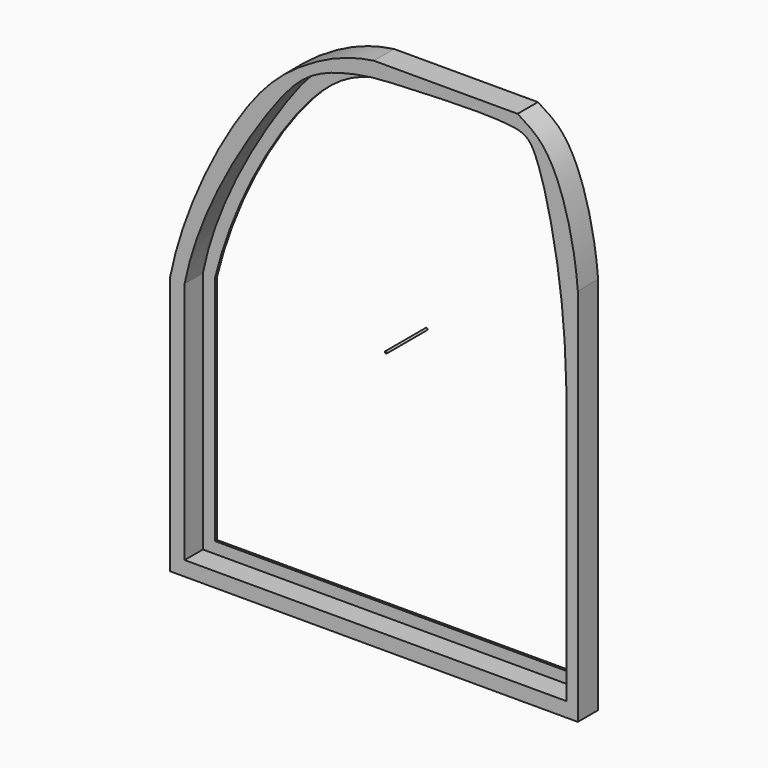
from build123d import *

# Parameters (mm, degrees)
F0_R     = 0.2107517129
F1_DEPTH = 10
F3_DEPTH = 5
F4_DEPTH = 0.5


with BuildPart() as f1:
    # F0 (on Front) → F1 (new body)
    with BuildSketch(Plane.XZ):
        Circle(F0_R)
    extrude(amount=F1_DEPTH)


with BuildPart() as f3:
    # F2 (on Front) → F3 (new body)
    with BuildSketch(Plane.XZ):
        with BuildLine():
            Line((21.9498877709, 46.5069999899), (-6.3801594079, 46.5069999899))
            add(Edge.make_bspline(
                [(-46.5855710208, -4.3176412582), (-44.0025745855, 8.8650835819), (-32.3669471438, 31.5826223404), (-20.8450996019, 41.430559805), (-11.9788710798, 45.7277535437), (-6.3801594079, 46.5069999899)],
                knots=[0, 0, 0, 0, 0.4471722481, 0.7226417186, 1, 1, 1, 1], degree=3))
            Line((-46.5855710208, -4.3176412582), (-46.5855710208, -55.1422825063))
            Line((-46.5855710208, -55.1422825063), (33.8252522051, -55.1422825063))
            Line((33.8252522051, -55.1422825063), (33.8252522051, 3.3716567512))
            add(Edge.make_bspline(
                [(33.8252522051, 3.4864664458), (33.8224510146, 3.4189701607), (33.823496077, 3.4012213221), (33.8252522051, 3.3716567512)],
                knots=[0.9714616128, 0.9714616128, 0.9714616128, 0.9714616128, 1, 1, 1, 1], degree=3))
            Line((33.8252522051, 3.4864664458), (33.8252522051, 19.6025110781))
            add(Edge.make_bspline(
                [(21.9498877709, 46.5069999899), (23.8964492564, 45.3404017708), (29.3341911452, 42.1357952335), (33.1026848595, 28.5809846581), (33.8252522051, 19.6025110781)],
                knots=[0, 0, 0, 0, 0.2303722913, 0.6333427683, 0.6333427683, 0.6333427683, 0.6333427683], degree=3))
        make_face()
        with BuildLine():
            Line((31.6210500896, -52.260261029), (-43.6766035855, -52.260261029))
            Line((-43.6766035855, -52.260261029), (-43.6766035855, -4.3176412582))
            add(Edge.make_bspline(
                [(-43.6766035855, -4.3176412582), (-41.0383021138, 9.0666906176), (-27.9398807539, 30.9156219348), (-18.7479844266, 41.3390835094), (-7.0085331076, 43.5985571671), (-2.215007715, 43.8020735184), (21.2993443911, 44.9657713637), (26.0800513958, 41.7197839808), (31.3102526714, 18.3624746495), (31.5930695379, 3.1075431018), (31.6210500896, -4.3176412582)],
                knots=[0, 0, 0, 0, 0.1942047864, 0.3092342936, 0.40822929, 0.4837495286, 0.6306580628, 0.7017097882, 0.8479049191, 1, 1, 1, 1], degree=3))
            Line((31.6210500896, -4.3176412582), (31.6210500896, -52.260261029))
        make_face(mode=Mode.SUBTRACT)
        with BuildLine():
            Line((33.8252522051, 3.3716567512), (33.8252522051, 3.4864664458))
            add(Edge.make_bspline(
                [(33.8252522051, 3.4864664458), (33.8224510146, 3.4189701607), (33.823496077, 3.4012213221), (33.8252522051, 3.3716567512)],
                knots=[0.9714616128, 0.9714616128, 0.9714616128, 0.9714616128, 1, 1, 1, 1], degree=3))
        make_face()
    extrude(amount=F3_DEPTH)

    # F2 (on Front) → F4 (join)
    with BuildSketch(Plane.XZ):
        with BuildLine():
            Line((-43.6766035855, -4.3176412582), (-43.6766035855, -52.260261029))
            Line((-43.6766035855, -52.260261029), (31.6210500896, -52.260261029))
            Line((31.6210500896, -52.260261029), (31.6210500896, -4.3176412582))
            add(Edge.make_bspline(
                [(-43.6766035855, -4.3176412582), (-41.0383021138, 9.0666906176), (-27.9398807539, 30.9156219348), (-18.7479844266, 41.3390835094), (-7.0085331076, 43.5985571671), (-2.215007715, 43.8020735184), (21.2993443911, 44.9657713637), (26.0800513958, 41.7197839808), (31.3102526714, 18.3624746495), (31.5930695379, 3.1075431018), (31.6210500896, -4.3176412582)],
                knots=[0, 0, 0, 0, 0.1942047864, 0.3092342936, 0.40822929, 0.4837495286, 0.6306580628, 0.7017097882, 0.8479049191, 1, 1, 1, 1], degree=3))
        make_face()
        with BuildLine():
            Line((29.4725894928, -50.028309226), (-41.2763357162, -50.028309226))
            Line((-41.2763357162, -50.028309226), (-41.2763357162, -4.3176412582))
            add(Edge.make_bspline(
                [(29.4725894928, -4.3176412582), (29.1241496967, 2.9787885737), (28.5454511929, 18.1687452905), (23.4164160844, 41.9172876242), (16.665337298, 42.2003372333), (-7.4096989865, 42.5160002908), (-22.9090094529, 36.1722681351), (-37.4855825891, 11.2133633357), (-41.2763357162, -4.3176412582)],
                knots=[0, 0, 0, 0, 0.1793175303, 0.3494515687, 0.4340680096, 0.6090858367, 0.7583926872, 1, 1, 1, 1], degree=3))
            Line((29.4725894928, -4.3176412582), (29.4725894928, -50.028309226))
        make_face(mode=Mode.SUBTRACT)
    extrude(amount=F4_DEPTH)


solid = Compound([f1.part, f3.part])
